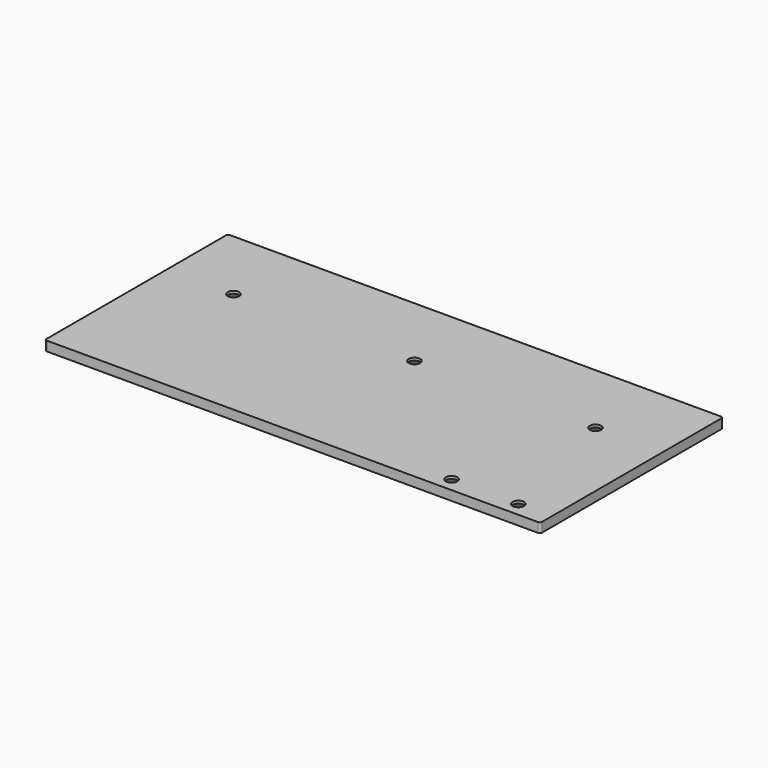
from build123d import *

# Parameters (mm, degrees)
F1_DEPTH       = 3.175
F2_D           = 3.7973
F2_CSINK_D     = 7.7978
F2_CSINK_ANGLE = 82


# Not quite as in the source:
# - a feature of the source that left no trace in its solid (it failed there, or was rolled back) is left out


with BuildPart() as f1:
    # F0 (on Top) → F1 (new body)
    with BuildSketch(Plane.XY):
        with BuildLine():
            Line((81.75625, 38.1), (-81.75625, 38.1))
            ThreePointArc((-81.75625, 38.1), (-82.3175160076, 37.8675160076), (-82.55, 37.30625))
            Line((-82.55, 37.30625), (-82.55, -37.30625))
            ThreePointArc((-82.55, -37.30625), (-82.3175160076, -37.8675160076), (-81.75625, -38.1))
            Line((-81.75625, -38.1), (81.75625, -38.1))
            ThreePointArc((81.75625, -38.1), (82.3175160076, -37.8675160076), (82.55, -37.30625))
            Line((82.55, -37.30625), (82.55, 37.30625))
            ThreePointArc((82.55, 37.30625), (82.3175160076, 37.8675160076), (81.75625, 38.1))
        make_face()
    extrude(amount=F1_DEPTH)

    # F2 (through all)
    with Locations(Plane(origin=(0, 0, 0), x_dir=(1, 0, 0), z_dir=(0, 0, -1))):
        with Locations((49.2125, 33.3375), (71.4375, 33.3375), (60.325, -12.7), (0, -12.7), (-60.325, -12.7)):
            CounterSinkHole(F2_D / 2, F2_CSINK_D / 2, counter_sink_angle=F2_CSINK_ANGLE)


solid = f1.part
